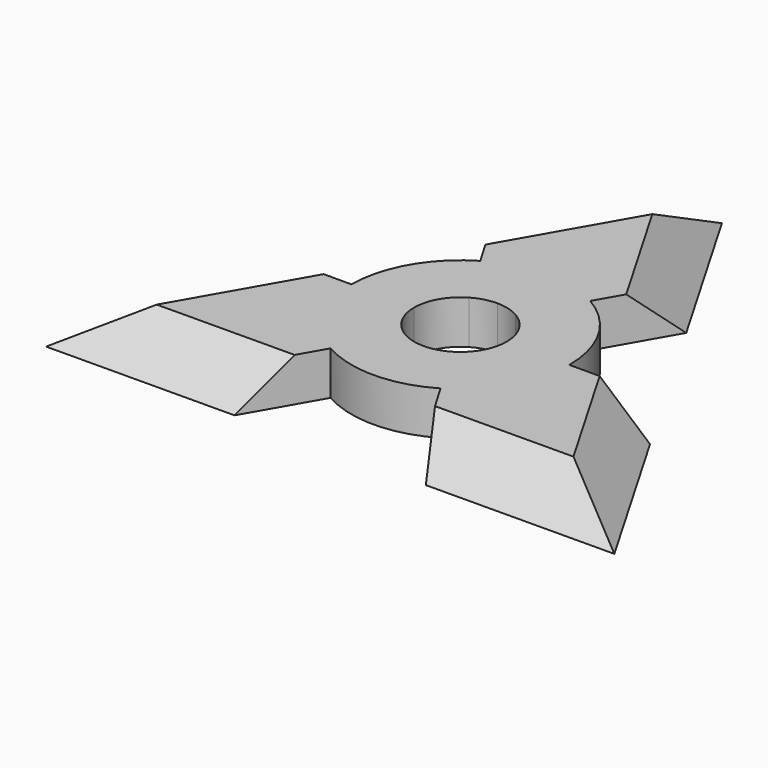
from build123d import *

# Parameters (mm, degrees)
F1_DEPTH = 5.08
F2_SIZE  = 5.07999


# Not quite as in the source:
# - a fillet or chamfer is up to 0.001 mm smaller than in the source, because OpenCascade refuses the exact size


with BuildPart() as f1:
    # F0 (on Top) → F1 (new body)
    with BuildSketch(Plane.XY):
        with BuildLine():
            ThreePointArc((-6.4398498965, 10.9461560975), (-3.3372007403, 12.2536970429), (0, 12.7))
            Line((0, 12.7), (0, 38.1))
            Line((0, 38.1), (-11.0489271221, 18.7804503105))
            Line((-11.0489271221, 18.7804503105), (-6.4398498965, 10.9461560975))
        make_face()
        with BuildLine():
            ThreePointArc((0, 12.7), (3.261881723, 12.2739613665), (6.304915, 11.0244295473))
            Line((6.304915, 11.0244295473), (10.9721234563, 19.185255))
            Line((10.9721234563, 19.185255), (0, 38.1))
            Line((0, 38.1), (0, 12.7))
        make_face()
        with BuildLine():
            ThreePointArc((-2.7338674235, 4.6469001683), (-1.4167200379, 5.2019819875), (0, 5.3914480674))
            Line((0, 5.3914480674), (0, 12.7))
            ThreePointArc((0, 12.7), (-3.3372007403, 12.2536970429), (-6.4398498965, 10.9461560975))
            Line((-6.4398498965, 10.9461560975), (-2.7338674235, 4.6469001683))
        make_face()
        with BuildLine():
            ThreePointArc((0, 5.3914480674), (1.3847453474, 5.2105846684), (2.6765843931, 4.6801290848))
            Line((2.6765843931, 4.6801290848), (6.304915, 11.0244295473))
            ThreePointArc((6.304915, 11.0244295473), (3.261881723, 12.2739613665), (0, 12.7))
            Line((0, 12.7), (0, 5.3914480674))
        make_face()
        with BuildLine():
            ThreePointArc((-5.3914480674, 0), (-4.6801290848, 2.6765843931), (-2.7338674235, 4.6469001683))
            Line((-2.7338674235, 4.6469001683), (-6.4398498965, 10.9461560975))
            ThreePointArc((-6.4398498965, 10.9461560975), (-11.0244295473, 6.304915), (-12.7, 0))
            Line((-12.7, 0), (-5.3914480674, 0))
        make_face()
        with BuildLine():
            ThreePointArc((2.6765843931, 4.6801290848), (4.6636025783, 2.7052769276), (5.3914480674, 0))
            Line((5.3914480674, 0), (12.7, 0))
            ThreePointArc((12.7, 0), (10.9855, 6.3725026285), (6.304915, 11.0244295473))
            Line((6.304915, 11.0244295473), (2.6765843931, 4.6801290848))
        make_face()
        with BuildLine():
            Line((-10.9461560975, -6.4398498965), (-4.6469001683, -2.7338674235))
            ThreePointArc((-4.6469001683, -2.7338674235), (-5.2019819875, -1.4167200379), (-5.3914480674, 0))
            Line((-5.3914480674, 0), (-12.7, 0))
            ThreePointArc((-12.7, 0), (-12.2536970429, -3.3372007403), (-10.9461560975, -6.4398498965))
        make_face()
        with BuildLine():
            Line((12.7, 0), (5.3914480674, 0))
            ThreePointArc((5.3914480674, 0), (5.2105846684, -1.3847453474), (4.6801290848, -2.6765843931))
            Line((4.6801290848, -2.6765843931), (11.0244295473, -6.304915))
            ThreePointArc((11.0244295473, -6.304915), (12.2739613665, -3.261881723), (12.7, 0))
        make_face()
        with BuildLine():
            Line((11.0244295473, -6.304915), (4.6801290848, -2.6765843931))
            ThreePointArc((4.6801290848, -2.6765843931), (3.835671013, -3.7888441699), (2.7338674235, -4.6469001683))
            Line((2.7338674235, -4.6469001683), (6.4398498965, -10.9461560975))
            ThreePointArc((6.4398498965, -10.9461560975), (9.0352390037, -8.9249345178), (11.0244295473, -6.304915))
        make_face()
        with BuildLine():
            Line((6.4398498965, -10.9461560975), (2.7338674235, -4.6469001683))
            ThreePointArc((2.7338674235, -4.6469001683), (0.0331115783, -5.3913463891), (-2.6765843931, -4.6801290848))
            Line((-2.6765843931, -4.6801290848), (-6.304915, -11.0244295473))
            ThreePointArc((-6.304915, -11.0244295473), (0.07799705, -12.6997604883), (6.4398498965, -10.9461560975))
        make_face()
        with BuildLine():
            ThreePointArc((-2.6765843931, -4.6801290848), (-3.7888441699, -3.835671013), (-4.6469001683, -2.7338674235))
            Line((-4.6469001683, -2.7338674235), (-10.9461560975, -6.4398498965))
            ThreePointArc((-10.9461560975, -6.4398498965), (-8.9249345178, -9.0352390037), (-6.304915, -11.0244295473))
            Line((-6.304915, -11.0244295473), (-2.6765843931, -4.6801290848))
        make_face()
        with BuildLine():
            Line((-32.8384682925, -19.3195496895), (-10.9461560975, -6.4398498965))
            ThreePointArc((-10.9461560975, -6.4398498965), (-12.2536970429, -3.3372007403), (-12.7, 0))
            Line((-12.7, 0), (-21.7895411704, 0))
            Line((-21.7895411704, 0), (-32.8384682925, -19.3195496895))
        make_face()
        with BuildLine():
            ThreePointArc((-6.304915, -11.0244295473), (-8.9249345178, -9.0352390037), (-10.9461560975, -6.4398498965))
            Line((-10.9461560975, -6.4398498965), (-32.8384682925, -19.3195496895))
            Line((-32.8384682925, -19.3195496895), (-10.9721234563, -19.185255))
            Line((-10.9721234563, -19.185255), (-6.304915, -11.0244295473))
        make_face()
        with BuildLine():
            Line((33.0732886418, -18.914745), (11.0244295473, -6.304915))
            ThreePointArc((11.0244295473, -6.304915), (9.0352390037, -8.9249345178), (6.4398498965, -10.9461560975))
            Line((6.4398498965, -10.9461560975), (11.2069438057, -19.0490396895))
            Line((11.2069438057, -19.0490396895), (33.0732886418, -18.914745))
        make_face()
        with BuildLine():
            Line((22.1011651855, 0), (12.7, 0))
            ThreePointArc((12.7, 0), (12.2739613665, -3.261881723), (11.0244295473, -6.304915))
            Line((11.0244295473, -6.304915), (33.0732886418, -18.914745))
            Line((33.0732886418, -18.914745), (22.1011651855, 0))
        make_face()
    extrude(amount=F1_DEPTH)

    # F2 (size 5.08 in the source; OpenCascade refuses exactly that, so slightly less here)
    f2_edges = [f1.edges().sort_by_distance(p)[0] for p in [
        (-5.524464, 28.440225, 5.08),
        (5.486062, 28.642628, 5.08),
        (-27.314005, -9.659775, 5.08),
        (-21.905296, -19.252402, 5.08),
        (22.140116, -18.981892, 5.08),
        (27.587227, -9.457373, 5.08),
    ]]
    chamfer(f2_edges, length=F2_SIZE)


solid = f1.part
